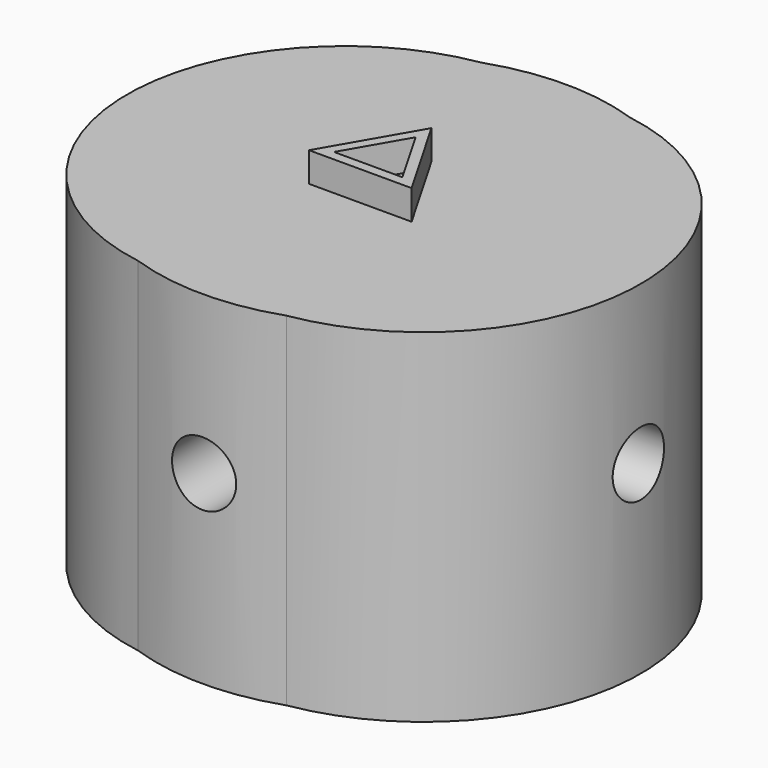
from build123d import *

# Parameters (mm, degrees)
F1_DEPTH       = 12
F3_R           = 3.25
F4_DEPTH       = 25
F4_DEPTH_BACK  = 25
F6_DEPTH       = 25
F12_DEPTH      = 22
F12_DEPTH_BACK = 12.75
F13_DEPTH      = 25
F13_DEPTH_BACK = 25
F14_R          = 3.25
F15_DEPTH      = 30
F15_DEPTH_BACK = 30
F16_R          = 2.125
F17_DEPTH      = 50
F18_DEPTH      = 3


# Not quite as in the source:
# - a feature of the source that left no trace in its solid (it failed there, or was rolled back) is left out
# - a feature names something its author has since deleted; it is built from what else it names


with BuildPart() as f1:
    # F0 (on Top) → F1 (new body)
    with BuildSketch(Plane.XY):
        with BuildLine():
            ThreePointArc((-11.87, 16.0966797819), (0, 20), (11.87, 16.0966797819))
            ThreePointArc((11.87, 16.0966797819), (0, 23), (-11.87, 16.0966797819))
        make_face()
        with BuildLine():
            ThreePointArc((-19.8751336077, 2.231381652), (-19.918584287, -11.5), (-8.0051336077, -18.3280614339))
            ThreePointArc((-8.0051336077, -18.3280614339), (-17.3205080757, -10), (-19.8751336077, 2.231381652))
        make_face()
        with BuildLine():
            ThreePointArc((19.8751336077, 2.231381652), (19.9687590019, 1.1174363173), (20, 0))
            ThreePointArc((20, 0), (16.7347344191, -10.9521077388), (8.0051336077, -18.3280614339))
            ThreePointArc((8.0051336077, -18.3280614339), (19.918584287, -11.5), (19.8751336077, 2.231381652))
        make_face()
        with BuildLine():
            ThreePointArc((8.0051336077, -18.3280614339), (16.7347344191, -10.9521077388), (20, 0))
            ThreePointArc((20, 0), (19.9687590019, 1.1174363173), (19.8751336077, 2.231381652))
            ThreePointArc((19.8751336077, 2.231381652), (17.3205080757, 10), (11.87, 16.0966797819))
            ThreePointArc((11.87, 16.0966797819), (0, 20), (-11.87, 16.0966797819))
            ThreePointArc((-11.87, 16.0966797819), (-17.3205080757, 10), (-19.8751336077, 2.231381652))
            ThreePointArc((-19.8751336077, 2.231381652), (-17.3205080757, -10), (-8.0051336077, -18.3280614339))
            ThreePointArc((-8.0051336077, -18.3280614339), (0, -20), (8.0051336077, -18.3280614339))
        make_face()
    extrude(amount=F1_DEPTH)

    # F3 (on offset) → F4 (cut, two sides)
    with BuildSketch(Plane.XZ) as f4_sk:
        with Locations((0, 6)):
            Circle(F3_R)
    extrude(amount=F4_DEPTH, mode=Mode.SUBTRACT)
    extrude(f4_sk.sketch, amount=-F4_DEPTH_BACK, mode=Mode.SUBTRACT)

    # F11 (on Top) → F12 (join, two sides)
    with BuildSketch(Plane.XY) as f12_sk:
        with BuildLine():
            ThreePointArc((7.5, -21.7428149052), (18.7283208003, -13.3510299228), (23, 0))
            ThreePointArc((23, 0), (18.7283208003, 13.3510299228), (7.5, 21.7428149052))
            ThreePointArc((7.5, 21.7428149052), (0, 23), (-7.5, 21.7428149052))
            ThreePointArc((-7.5, 21.7428149052), (-23, 0), (-7.5, -21.7428149052))
            ThreePointArc((-7.5, -21.7428149052), (0, -23), (7.5, -21.7428149052))
        make_face()
        with BuildLine():
            ThreePointArc((-7.5, -21.7428149052), (-23, 0), (-7.5, 21.7428149052))
            ThreePointArc((-7.5, 21.7428149052), (-26, 0), (-7.5, -21.7428149052))
        make_face()
        with BuildLine():
            ThreePointArc((7.5, 21.7428149052), (18.7283208003, 13.3510299228), (23, 0))
            ThreePointArc((23, 0), (18.7283208003, -13.3510299228), (7.5, -21.7428149052))
            ThreePointArc((7.5, -21.7428149052), (26, 0), (7.5, 21.7428149052))
        make_face()
    extrude(amount=F12_DEPTH)
    extrude(f12_sk.sketch, amount=-F12_DEPTH_BACK)

    # F3 (on offset) → F13 (cut, two sides)
    with BuildSketch(Plane.XZ) as f13_sk:
        with Locations((0, 6)):
            Circle(F3_R)
    extrude(amount=-F13_DEPTH, mode=Mode.SUBTRACT)
    extrude(f13_sk.sketch, amount=F13_DEPTH_BACK, mode=Mode.SUBTRACT)

    # F14 (on Right) → F15 (cut, two sides)
    with BuildSketch(Plane.YZ) as f15_sk:
        with Locations((0, 6)):
            Circle(F14_R)
    extrude(amount=-F15_DEPTH, mode=Mode.SUBTRACT)
    extrude(f15_sk.sketch, amount=F15_DEPTH_BACK, mode=Mode.SUBTRACT)

    # F16 (on face) → F17 (cut)
    with BuildSketch(Plane(origin=(0, 0, -12.75), x_dir=(1, 0, 0), z_dir=(0, 0, -1))):
        Circle(F16_R)
    extrude(amount=-F17_DEPTH, mode=Mode.SUBTRACT)

    # F16 (on face) → F18 (cut)
    with BuildSketch(Plane(origin=(0, 0, -12.75), x_dir=(1, 0, 0), z_dir=(0, 0, -1))):
        Polygon((-0.2451741669, -4.3231804991), (3.6213970539, -2.3739173065), (3.8665712208, 1.9492631926), (0.2451741669, 4.3231804991), (-3.6213970539, 2.3739173065), (-3.8665712208, -1.9492631926), align=None)
        Circle(F16_R, mode=Mode.SUBTRACT)
    extrude(amount=-F18_DEPTH, mode=Mode.SUBTRACT)


with BuildPart() as f6:
    # F5 (on Top) → F6 (new body)
    with BuildSketch(Plane.XY):
        Polygon((-5.1961524227, -3), (5.1961524227, -3), (0, 6), align=None)
        Polygon((0, 4), (3.4641016151, -2), (-3.4641016151, -2), align=None, mode=Mode.SUBTRACT)
    extrude(amount=F6_DEPTH)


solid = Compound([f1.part, f6.part])
